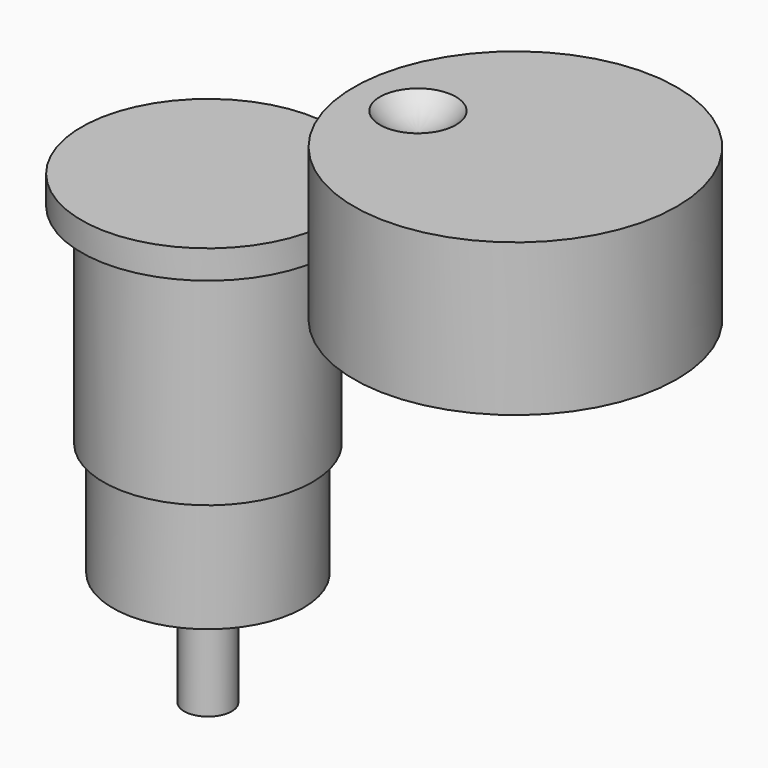
from build123d import *

# Parameters (mm, degrees)
F0_R     = 3.175
F1_DEPTH = 58.42
F0_R_2   = 12.7
F2_DEPTH = 43.18
F0_R_3   = 13.97
F3_DEPTH = 27.94
F0_R_4   = 16.891
F4_DEPTH = 3.81
F0_R_5   = 21.59
F5_DEPTH = 20.32
F6_R     = 5.08
F7_DEPTH = 2.54


# Not quite as in the source:
# - a fillet or chamfer that OpenCascade refuses, or shapes differently, is made with other operations: its cross-section is extruded or revolved along the edge and cut away or added


with BuildPart() as f1:
    # F0 (on Top) → F1 (new body)
    with BuildSketch(Plane.XY):
        Circle(F0_R)
    extrude(amount=-F1_DEPTH)

    # F0 (on Top) → F2 (join)
    with BuildSketch(Plane.XY):
        Circle(F0_R_2)
        Circle(F0_R, mode=Mode.SUBTRACT)
    extrude(amount=-F2_DEPTH)

    # F0 (on Top) → F3 (join)
    with BuildSketch(Plane.XY):
        Circle(F0_R_3)
        Circle(F0_R_2, mode=Mode.SUBTRACT)
    extrude(amount=-F3_DEPTH)

    # F0 (on Top) → F4 (join)
    with BuildSketch(Plane.XY):
        Circle(F0_R_4)
        Circle(F0_R_3, mode=Mode.SUBTRACT)
        Circle(F0_R_3)
        Circle(F0_R_2, mode=Mode.SUBTRACT)
        Circle(F0_R_2)
        Circle(F0_R, mode=Mode.SUBTRACT)
        Circle(F0_R)
    extrude(amount=F4_DEPTH)


with BuildPart() as f5:
    # F0 (on Top) → F5 (new body)
    with BuildSketch(Plane.XY):
        with Locations((41.0842709243, 0)):
            Circle(F0_R_5)
    extrude(amount=F5_DEPTH)

    # F6 (on face) → F7 (cut)
    with BuildSketch(Plane.XY.offset(20.32)):
        with Locations((28.0622877181, 0)):
            Circle(F6_R)
    extrude(amount=-F7_DEPTH, mode=Mode.SUBTRACT)

    # F8: fillet of radius 6.223 on 1 edges, made by hand

    # F8_s1 → F8_t2 (revolve)
    with BuildSketch(Plane.XZ):
        with BuildLine():
            ThreePointArc((33.1422877181, 20.32), (30.9374544728, 18.4511967794), (28.1261896329, 17.78))
            Line((28.1261896329, 17.78), (33.1422877181, 17.78))
            Line((33.1422877181, 17.78), (33.1422877181, 20.32))
        make_face()
    revolve(axis=Axis((28.0622877181, 0, 17.78), (0, 0, 1)))


solid = Compound([f1.part, f5.part])
